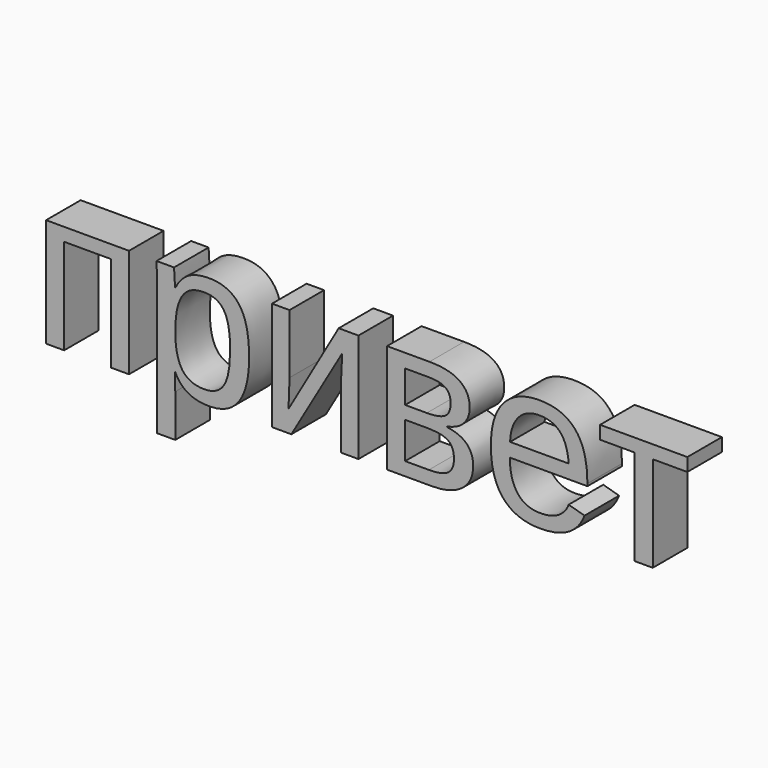
from build123d import *

# Parameters (mm, degrees)
F0_TEXT_SIZE = 120.9920479192
F1_DEPTH     = 25.4


# Not quite as in the source:
# - Text() gives the source's letters only with a copy of the font that has no kerning and outlines rounded to 1/6400 em; it was checked with that copy


with BuildPart() as f1:
    # F0 (on Front) → F1 (new body)
    with BuildSketch(Plane.XZ):
        with Locations((-55.1436319947, -57.1891590953)):
            Text('привет', F0_TEXT_SIZE, font='Arimo', text_align=(TextAlign.LEFT, TextAlign.BOTTOM))
    extrude(amount=F1_DEPTH)


solid = f1.part
